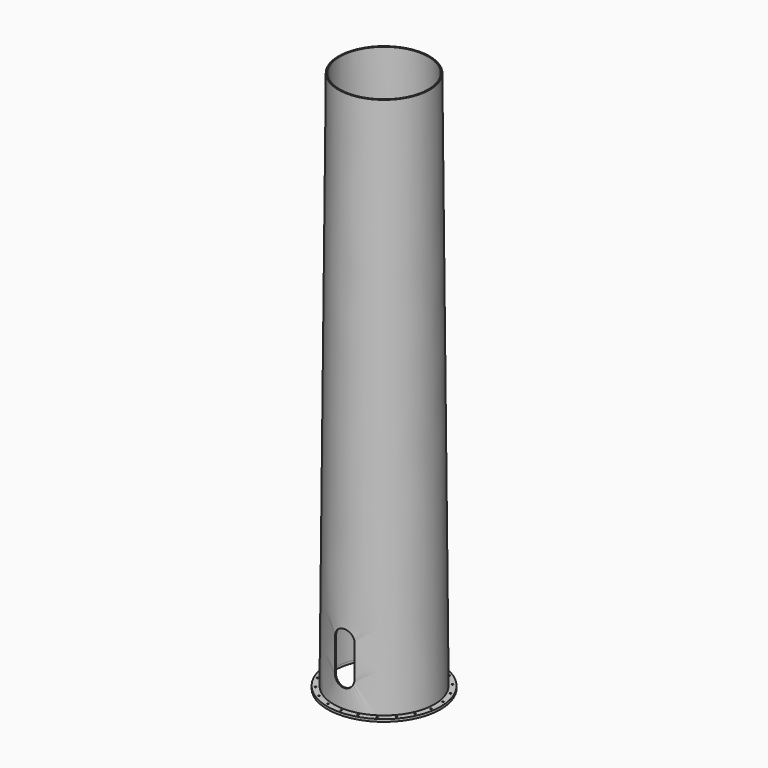
from build123d import *

# Parameters (mm, degrees)
F2_R            = 30
F3_DEPTH        = 100
F3_COPIES_COUNT = 22
F5_DEPTH        = 2500


# Not quite as in the source:
# - a pattern or mirror of a feature is missing from the dataset's text; its kind, count and spacing are read off the source's solid


with BuildPart() as f1:
    # F0 (on Front) → F1 (revolve)
    with BuildSketch(Plane.XZ):
        Polygon((2000, 100), (2000, 0), (2300, 0), (2300, 100), (2050.0020849839, 100), (1850.0020849839, 22000), (1800, 22000), align=None)
    revolve(axis=Axis((0, 0, 11000), (0, 0, 1)))

    # F2 (on face) → F3 (cut, through all)
    with BuildSketch(Plane(origin=(0, 0, 0), x_dir=(1, 0, 0), z_dir=(0, 0, -1))):
        with Locations((0, -2175)):
            Circle(F2_R)
    f3 = extrude(amount=-F3_DEPTH, mode=Mode.SUBTRACT)

    # F3_copies: F3 ×22 about axis
    f3_copies_axis = Axis((0, 0, 0), (0, 0, 1))
    for i in range(1, F3_COPIES_COUNT):
        add(f3.rotate(f3_copies_axis, i * 360 / F3_COPIES_COUNT), mode=Mode.SUBTRACT)

    # F4 (on Front) → F5 (cut)
    with BuildSketch(Plane.XZ):
        with BuildLine():
            ThreePointArc((-400, 1250), (0, 850), (400, 1250))
            Line((400, 1250), (400, 2550))
            ThreePointArc((400, 2550), (0, 2950), (-400, 2550))
            Line((-400, 2550), (-400, 1250))
        make_face()
    extrude(amount=F5_DEPTH, mode=Mode.SUBTRACT)


solid = f1.part
